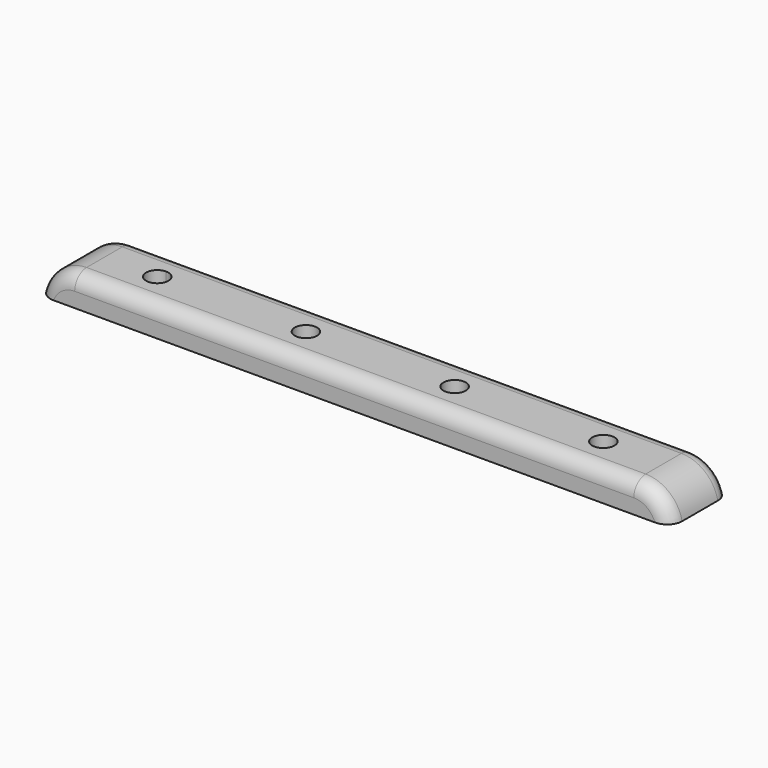
from build123d import *

# Parameters (mm, degrees)
F0_W        = 85
F0_H        = 10
F0_R        = 1.5
F1_DEPTH    = 4
F2_T1_DEPTH = 34.4948974279
F3_R        = 2


# Not quite as in the source:
# - a fillet or chamfer that OpenCascade refuses, or shapes differently, is made with other operations: its cross-section is extruded or revolved along the edge and cut away or added


with BuildPart() as f1:
    # F0 (on Top) → F1 (new body)
    with BuildSketch(Plane.XY):
        with Locations((5.8581340313, 5)):
            Rectangle(F0_W, F0_H)
        with BuildLine():
            ThreePointArc((-24.6418659687, 6.5), (-23.5812057969, 6.0606601718), (-23.1418659687, 5))
            ThreePointArc((-23.1418659687, 5), (-23.5812057969, 3.9393398282), (-24.6418659687, 3.5))
            ThreePointArc((-24.6418659687, 3.5), (-26.1418659687, 5), (-24.6418659687, 6.5))
        make_face(mode=Mode.SUBTRACT)
        with Locations((-4.6418659687, 5)):
            Circle(F0_R, mode=Mode.SUBTRACT)
        with Locations((15.3581340313, 5)):
            Circle(F0_R, mode=Mode.SUBTRACT)
        with Locations((35.3581340313, 5)):
            Circle(F0_R, mode=Mode.SUBTRACT)
    extrude(amount=F1_DEPTH)

    # F2: fillet of radius 5 on 2 edges, made by hand

    # F2_s2 → F2_t1 (cut)
    with BuildSketch(Plane.XZ.offset(-22.2474487139)):
        with BuildLine():
            ThreePointArc((-31.7428864831, 4), (-34.9051641433, 2.8729833462), (-36.6418659687, 0))
            Line((-36.6418659687, 0), (-36.6418659687, 4))
            Line((-36.6418659687, 4), (-31.7428864831, 4))
        make_face()
        with BuildLine():
            ThreePointArc((43.4591545457, 4), (46.6214322059, 2.8729833462), (48.3581340313, 0))
            Line((48.3581340313, 0), (48.3581340313, 4))
            Line((48.3581340313, 4), (43.4591545457, 4))
        make_face()
    extrude(amount=F2_T1_DEPTH, mode=Mode.SUBTRACT)

    # F3
    f3_edges = [f1.edges().sort_by_distance(p)[0] for p in [
        (5.858134, 10, 4),
        (5.858134, 0, 4),
        (-34.905164, 10, 2.872983),
        (46.621432, 10, 2.872983),
        (-34.905164, 0, 2.872983),
        (46.621432, 0, 2.872983),
    ]]
    fillet(f3_edges, radius=F3_R)


solid = f1.part
